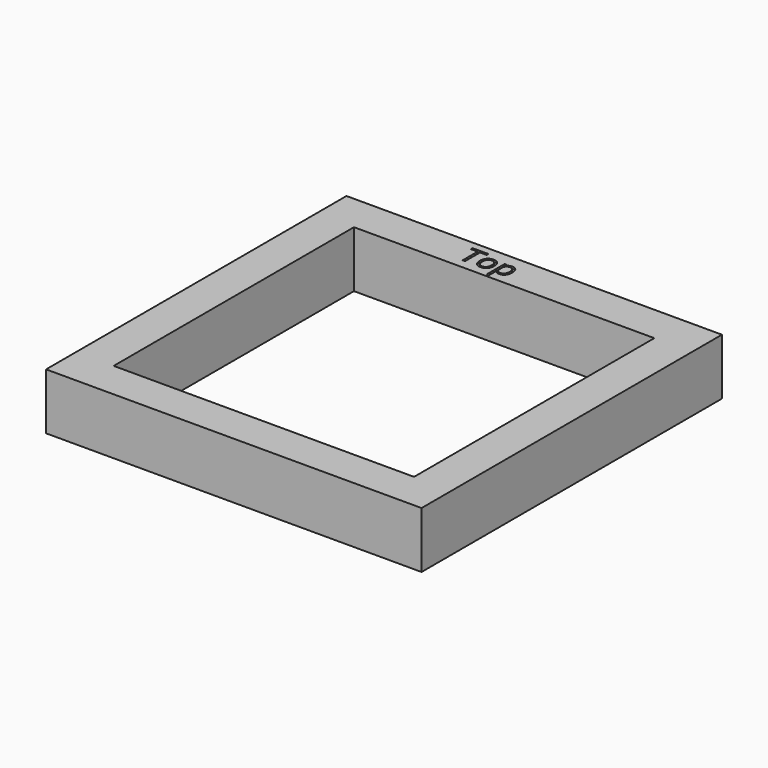
from build123d import *

# Parameters (mm, degrees)
F0_W         = 100
F0_H         = 100
F0_W_2       = 80
F0_H_2       = 80
F1_DEPTH     = 15
F3_TEXT_SIZE = 7.7996196018
F4_DEPTH     = 0.5
F5_TEXT_SIZE = 7.1486044261
F6_DEPTH     = 0.5


# Not quite as in the source:
# - Text() gives the source's letters only with a copy of the font that has no kerning and outlines rounded to 1/6400 em; it was checked with that copy


with BuildPart() as f1:
    # F0 (on Top) → F1 (new body)
    with BuildSketch(Plane.XY):
        Rectangle(F0_W, F0_H)
        Rectangle(F0_W_2, F0_H_2, mode=Mode.SUBTRACT)
    extrude(amount=F1_DEPTH)

    # F3 (on offset) → F4 (cut)
    with BuildSketch(Plane.XY.offset(15)):
        with Locations((-14.8747246712, 42.4710996449)):
            Text('Top', F3_TEXT_SIZE, font='Open Sans', text_align=(TextAlign.LEFT, TextAlign.BOTTOM))
    extrude(amount=-F4_DEPTH, mode=Mode.SUBTRACT)

    # F5 (on Top) → F6 (cut)
    with BuildSketch(Plane.XY):
        with Locations((-12.2223906219, 41.4127297699)):
            Text('Bottom', F5_TEXT_SIZE, font='Open Sans', text_align=(TextAlign.LEFT, TextAlign.BOTTOM))
    extrude(amount=F6_DEPTH, mode=Mode.SUBTRACT)


solid = f1.part
